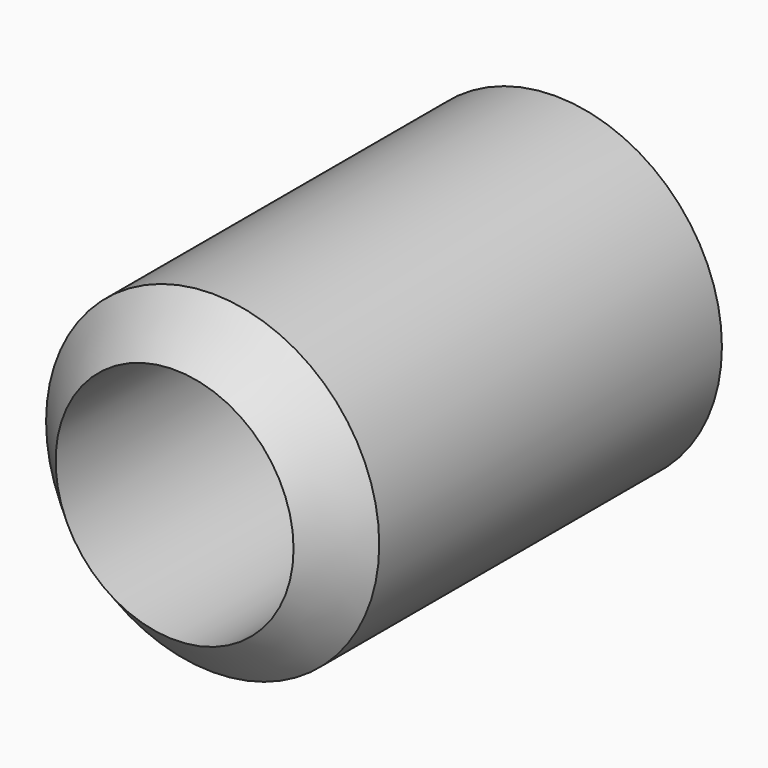
from build123d import *

# Parameters (mm, degrees)
F0_R     = 7
F0_R_2   = 5
F1_DEPTH = 20
F2_SIZE  = 1.99999


# Not quite as in the source:
# - a fillet or chamfer is up to 0.001 mm smaller than in the source, because OpenCascade refuses the exact size


with BuildPart() as f1:
    # F0 (on Front) → F1 (new body)
    with BuildSketch(Plane.XZ):
        Circle(F0_R)
        Circle(F0_R_2, mode=Mode.SUBTRACT)
    extrude(amount=F1_DEPTH)

    # F2 (size 2 in the source; OpenCascade refuses exactly that, so slightly less here)
    f2_edges = [f1.edges().sort_by_distance(p)[0] for p in [
        (-7, -20, 0),
    ]]
    chamfer(f2_edges, length=F2_SIZE)


solid = f1.part
